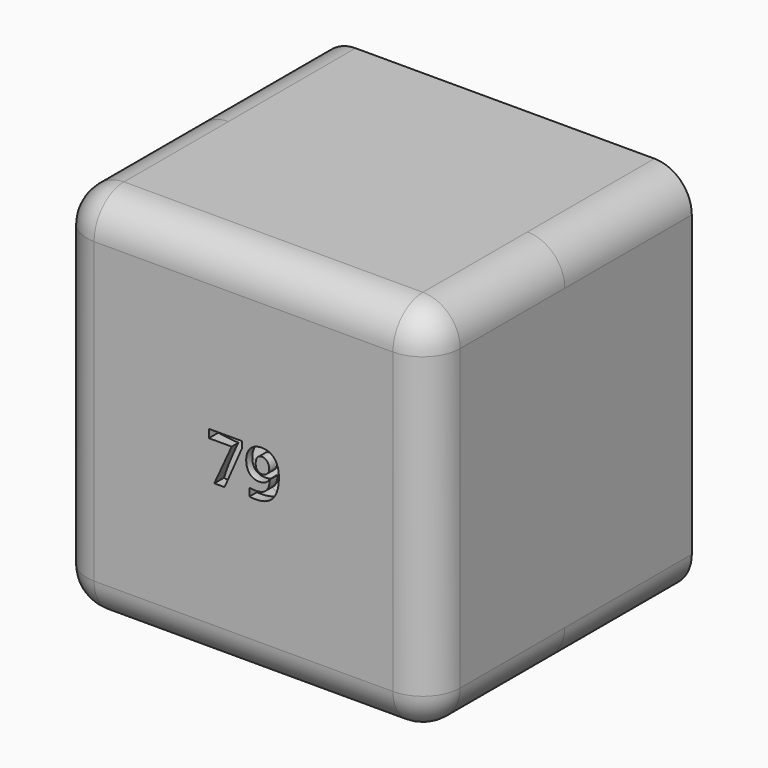
from build123d import *

# Parameters (mm, degrees)
F0_W         = 50.8
F0_H         = 50.8
F0_R         = 21.59
F1_DEPTH     = 22.86
F4_R         = 5.08
F5_TEXT_SIZE = 8.8194444444
F6_DEPTH     = 25.4
F7_R         = 21.844
F8_DEPTH     = 21.59


# Not quite as in the source:
# - Text() gives the source's letters only with a copy of the font that has no kerning and outlines rounded to 1/6400 em; it was checked with that copy


with BuildPart() as f1:
    # F0 (on Front) → F1 (new body)
    with BuildSketch(Plane.XZ):
        Rectangle(F0_W, F0_H)
        Circle(F0_R, mode=Mode.SUBTRACT)
        Circle(F0_R)
    extrude(amount=F1_DEPTH)

    # F2 (on Right) → F3 (revolve, cut)
    with BuildSketch(Plane.YZ):
        with BuildLine():
            Line((0, -21.844), (0, 0))
            Line((0, 0), (-21.844, 0))
            ThreePointArc((-21.844, 0), (-15.4460405282, -15.4460405282), (0, -21.844))
        make_face()
    revolve(axis=Axis((0, -10.922, 0), (0, -1, 0)), mode=Mode.SUBTRACT)

    # F4
    f4_edges = [f1.edges().sort_by_distance(p)[0] for p in [
        (0, -22.86, -25.4),
        (25.4, -22.86, 0),
        (0, -22.86, 25.4),
        (-25.4, -22.86, 0),
        (-25.4, -11.43, 25.4),
        (25.4, -11.43, 25.4),
        (-25.4, -11.43, -25.4),
        (25.4, -11.43, -25.4),
    ]]
    fillet(f4_edges, radius=F4_R)

    # F5 (on face) → F6 (cut)
    with BuildSketch(Plane.XZ.offset(22.86)):
        with Locations((-4.9516963397, -3.3079943313)):
            Text('79', F5_TEXT_SIZE, font='Open Sans', font_style=FontStyle.BOLD, text_align=(TextAlign.LEFT, TextAlign.BOTTOM))
    extrude(amount=-F6_DEPTH, mode=Mode.SUBTRACT)

    # F7 (on face) → F8 (join)
    with BuildSketch(Plane(origin=(0, 0, 0), x_dir=(-1, 0, 0), z_dir=(0, 1, 0))):
        with BuildLine():
            ThreePointArc((-25.4, -20.32), (-23.9121024484, -23.9121024484), (-20.32, -25.4))
            Line((-20.32, -25.4), (20.32, -25.4))
            ThreePointArc((20.32, -25.4), (23.9121024484, -23.9121024484), (25.4, -20.32))
            Line((25.4, -20.32), (25.4, 20.32))
            ThreePointArc((25.4, 20.32), (23.9121024484, 23.9121024484), (20.32, 25.4))
            Line((20.32, 25.4), (-20.32, 25.4))
            ThreePointArc((-20.32, 25.4), (-23.9121024484, 23.9121024484), (-25.4, 20.32))
            Line((-25.4, 20.32), (-25.4, -20.32))
        make_face()
        Circle(F7_R, mode=Mode.SUBTRACT)
    extrude(amount=F8_DEPTH)


solid = f1.part
